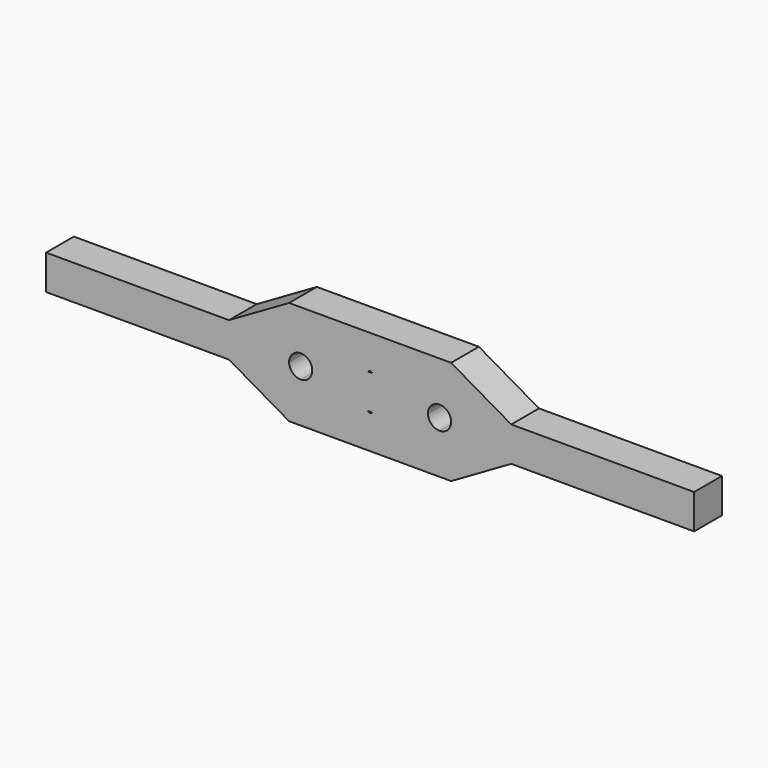
from build123d import *

# Parameters (mm, degrees)
F1_DEPTH = 19.05


with BuildPart() as f1:
    # F0 (on Front) → F1 (new body)
    with BuildSketch(Plane.XZ):
        Polygon((-80.3030704341, -65.7893445744), (-180.6575025499, -65.7893445744), (-180.6575025499, -84.8393445744), (-80.3030704341, -84.8393445744), (-47.3075025499, -84.8393445744), (-47.3075025499, -75.3143445744), (-47.3075025499, -65.7893445744), align=None)
        Polygon((-47.3075025499, -46.7393445744), (-80.3030704341, -65.7893445744), (-47.3075025499, -65.7893445744), align=None)
        Polygon((-47.3075025499, -46.7393445744), (-47.3075025499, -65.7893445744), (-40.9575025499, -65.7893445744), (-34.6075025499, -65.7893445744), (-34.6075025499, -46.7393445744), align=None)
        with BuildLine():
            Line((-40.9575025499, -65.7893445744), (-47.3075025499, -65.7893445744))
            Line((-47.3075025499, -65.7893445744), (-47.3075025499, -75.3143445744))
            ThreePointArc((-47.3075025499, -75.3143445744), (-45.4476306104, -70.8242165139), (-40.9575025499, -68.9643445744))
            Line((-40.9575025499, -68.9643445744), (-40.9575025499, -65.7893445744))
        make_face()
        Polygon((-47.3075025499, -84.8393445744), (-80.3030704341, -84.8393445744), (-47.3075025499, -103.8893445744), align=None)
        with BuildLine():
            Line((-34.6075025499, -65.7893445744), (-40.9575025499, -65.7893445744))
            Line((-40.9575025499, -65.7893445744), (-40.9575025499, -68.9643445744))
            ThreePointArc((-40.9575025499, -68.9643445744), (-36.4673744894, -70.8242165139), (-34.6075025499, -75.3143445744))
            Line((-34.6075025499, -75.3143445744), (-34.6075025499, -65.7893445744))
        make_face()
        with BuildLine():
            ThreePointArc((-40.9575025499, -81.6643445744), (-45.4476306104, -79.8044726349), (-47.3075025499, -75.3143445744))
            Line((-47.3075025499, -75.3143445744), (-47.3075025499, -84.8393445744))
            Line((-47.3075025499, -84.8393445744), (-43.3831779935, -84.8393445744))
            Line((-43.3831779935, -84.8393445744), (-40.9575025499, -84.8393445744))
            Line((-40.9575025499, -84.8393445744), (-40.9575025499, -81.6643445744))
        make_face()
        Polygon((-2.8575025499, -65.0702156212), (-34.6075025499, -46.7393445744), (-34.6075025499, -65.7893445744), (-4.1030704341, -65.7893445744), align=None)
        Polygon((28.8924974501, -46.7393445744), (-34.6075025499, -46.7393445744), (-2.8575025499, -65.0702156212), align=None)
        Polygon((-43.3831779935, -84.8393445744), (-47.3075025499, -84.8393445744), (-47.3075025499, -103.8893445744), (-34.6075025499, -103.8893445744), (-34.6075025499, -84.8393445744), (-40.9575025499, -84.8393445744), align=None)
        Polygon((-4.1030704341, -65.7893445744), (-34.6075025499, -65.7893445744), (-34.6075025499, -75.3143445744), (-34.6075025499, -84.8393445744), (-4.1030704341, -84.8393445744), (-2.8575025499, -84.8393445744), (-2.8575025499, -65.7893445744), align=None)
        with BuildLine():
            ThreePointArc((-34.6075025499, -75.3143445744), (-36.4673744894, -79.8044726349), (-40.9575025499, -81.6643445744))
            Line((-40.9575025499, -81.6643445744), (-40.9575025499, -84.8393445744))
            Line((-40.9575025499, -84.8393445744), (-34.6075025499, -84.8393445744))
            Line((-34.6075025499, -84.8393445744), (-34.6075025499, -75.3143445744))
        make_face()
        Polygon((28.8924974501, -46.7393445744), (-2.8575025499, -65.0702156212), (-1.6119346657, -65.7893445744), (28.8924974501, -65.7893445744), align=None)
        Polygon((41.5924974501, -46.7393445744), (28.8924974501, -46.7393445744), (28.8924974501, -65.7893445744), (35.2424974501, -65.7893445744), (41.5924974501, -65.7893445744), align=None)
        Polygon((-34.6075025499, -84.8393445744), (-34.6075025499, -103.8893445744), (-2.8575025499, -85.5584735276), (-4.1030704341, -84.8393445744), align=None)
        Polygon((-2.8575025499, -85.5584735276), (-34.6075025499, -103.8893445744), (28.8924974501, -103.8893445744), align=None)
        Polygon((28.8924974501, -65.7893445744), (-1.6119346657, -65.7893445744), (-2.8575025499, -65.7893445744), (-2.8575025499, -84.8393445744), (-1.6119346657, -84.8393445744), (28.8924974501, -84.8393445744), (28.8924974501, -75.3143445744), align=None)
        Polygon((74.5880653343, -65.7893445744), (41.5924974501, -46.7393445744), (41.5924974501, -65.7893445744), align=None)
        with BuildLine():
            Line((35.2424974501, -65.7893445744), (28.8924974501, -65.7893445744))
            Line((28.8924974501, -65.7893445744), (28.8924974501, -75.3143445744))
            ThreePointArc((28.8924974501, -75.3143445744), (30.7523693896, -70.8242165139), (35.2424974501, -68.9643445744))
            Line((35.2424974501, -68.9643445744), (35.2424974501, -65.7893445744))
        make_face()
        Polygon((-1.6119346657, -84.8393445744), (-2.8575025499, -85.5584735276), (28.8924974501, -103.8893445744), (28.8924974501, -84.8393445744), align=None)
        Polygon((28.8924974501, -84.8393445744), (28.8924974501, -103.8893445744), (41.5924974501, -103.8893445744), (41.5924974501, -84.8393445744), (35.2424974501, -84.8393445744), align=None)
        with BuildLine():
            Line((41.5924974501, -75.3143445744), (41.5924974501, -65.7893445744))
            Line((41.5924974501, -65.7893445744), (35.2424974501, -65.7893445744))
            Line((35.2424974501, -65.7893445744), (35.2424974501, -68.9643445744))
            ThreePointArc((35.2424974501, -68.9643445744), (39.7326255106, -70.8242165139), (41.5924974501, -75.3143445744))
        make_face()
        Polygon((74.5880653343, -65.7893445744), (41.5924974501, -65.7893445744), (41.5924974501, -75.3143445744), (41.5924974501, -84.8393445744), (74.5880653343, -84.8393445744), (174.9424974501, -84.8393445744), (174.9424974501, -65.7893445744), align=None)
        with BuildLine():
            ThreePointArc((35.2424974501, -81.6643445744), (30.7523693896, -79.8044726349), (28.8924974501, -75.3143445744))
            Line((28.8924974501, -75.3143445744), (28.8924974501, -84.8393445744))
            Line((28.8924974501, -84.8393445744), (35.2424974501, -84.8393445744))
            Line((35.2424974501, -84.8393445744), (35.2424974501, -81.6643445744))
        make_face()
        Polygon((41.5924974501, -84.8393445744), (41.5924974501, -103.8893445744), (74.5880653343, -84.8393445744), align=None)
        with BuildLine():
            Line((41.5924974501, -84.8393445744), (41.5924974501, -75.3143445744))
            ThreePointArc((41.5924974501, -75.3143445744), (39.7326255106, -79.8044726349), (35.2424974501, -81.6643445744))
            Line((35.2424974501, -81.6643445744), (35.2424974501, -84.8393445744))
            Line((35.2424974501, -84.8393445744), (41.5924974501, -84.8393445744))
        make_face()
    extrude(amount=F1_DEPTH)


solid = f1.part
